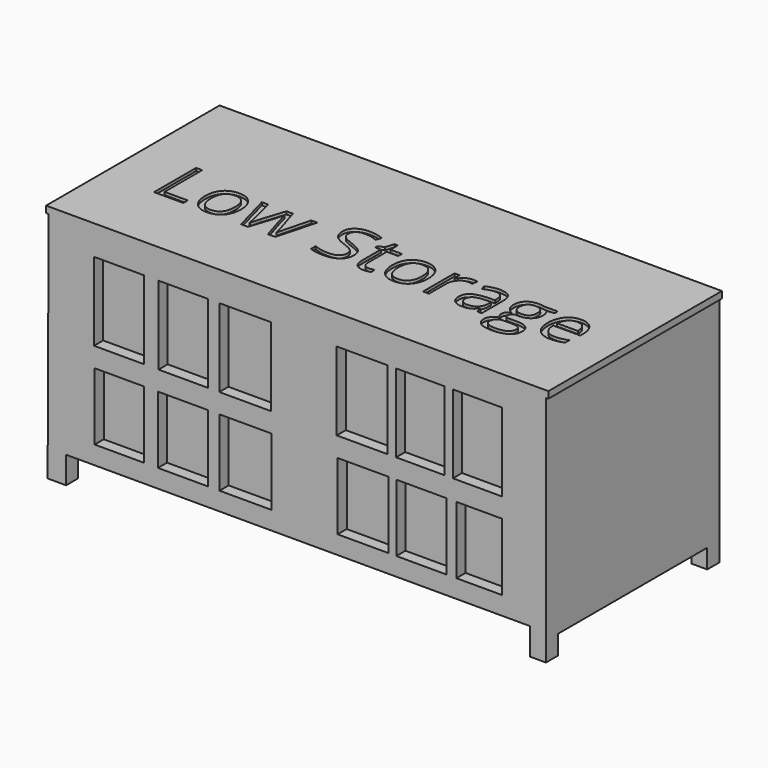
from build123d import *

# Parameters (mm, degrees)
F0_W         = 1117.6
F0_H         = 482.6
F1_DEPTH     = 533.4
F2_W         = 1032.1243926883
F2_H         = 59.8569884896
F3_DEPTH     = 482.601
F4_W         = 415.7167449594
F4_H         = 42.7146777511
F5_DEPTH     = 1117.601
F6_W         = 111.7840632796
F6_H         = 174.2089092731
F6_W_2       = 110.3323251009
F6_W_3       = 114.6875321865
F6_W_4       = 108.8805794716
F6_W_5       = 107.4288487434
F6_W_6       = 113.2358312607
F6_H_2       = 149.5293006301
F6_W_7       = 111.784055829
F6_W_8       = 116.139292717
F6_W_9       = 101.6219258308
F6_W_10      = 111.7841005325
F6_W_11      = 113.235771656
F7_DEPTH     = 25.4
F8_TEXT_SIZE = 163.7518405914
F9_DEPTH     = 6.35
F10_W        = 5.4096342087
F10_H        = 518.5263156891
F11_DEPTH    = 482.6010001


# Not quite as in the source:
# - a length typed as a fraction of an inch, garbled in the dataset ("3 / 203.2 mm" for 3/8 in), is restored
# - Text() gives the source's letters only with a copy of the font that has no kerning and outlines rounded to 1/6400 em; it was checked with that copy


with BuildPart() as f1:
    # F0 (on Top) → F1 (new body)
    with BuildSketch(Plane.XY):
        with Locations((558.8, 241.3)):
            Rectangle(F0_W, F0_H)
    extrude(amount=F1_DEPTH)

    # F2 (on face) → F3 (cut, through all)
    with BuildSketch(Plane.XZ):
        with Locations((560.7183612883, 29.9284942448)):
            Rectangle(F2_W, F2_H)
    extrude(amount=-F3_DEPTH, mode=Mode.SUBTRACT)

    # F4 (on face) → F5 (cut, through all)
    with BuildSketch(Plane.YZ.offset(1117.6)):
        with Locations((240.7026998699, 21.3573388755)):
            Rectangle(F4_W, F4_H)
    extrude(amount=-F5_DEPTH, mode=Mode.SUBTRACT)

    # F6 (on face) → F7 (cut)
    with BuildSketch(Plane.XZ):
        with Locations((162.4746061862, 380.6616812944)):
            Rectangle(F6_W, F6_H)
        with Locations((305.4711148143, 380.6616812944)):
            Rectangle(F6_W_2, F6_H)
        with Locations((442.6606446505, 380.6616812944)):
            Rectangle(F6_W_3, F6_H)
        with Locations((959.4804644585, 380.6616812944)):
            Rectangle(F6_W_4, F6_H)
        with Locations((832.4531316757, 380.6616812944)):
            Rectangle(F6_W_5, F6_H)
        with Locations((703.2481729984, 380.6616812944)):
            Rectangle(F6_W_6, F6_H)
        with Locations((163.2005050778, 175.2402968705)):
            Rectangle(F6_W_2, F6_H_2)
        with Locations((304.7452494502, 175.2402968705)):
            Rectangle(F6_W_7, F6_H_2)
        with Locations((443.9914307247, 175.2402968705)):
            Rectangle(F6_W_8, F6_H_2)
        with Locations((963.7147268901, 175.2402968705)):
            Rectangle(F6_W_9, F6_H_2)
        with Locations((835.2356335769, 175.2402968705)):
            Rectangle(F6_W_10, F6_H_2)
        with Locations((705.3048095355, 175.2402968705)):
            Rectangle(F6_W_11, F6_H_2)
    extrude(amount=-F7_DEPTH, mode=Mode.SUBTRACT)

    # F8 (on face) → F9 (cut)
    with BuildSketch(Plane.XY.offset(533.4)):
        with Locations((98.7801775336, 156.6599458456)):
            Text('Low Storage', F8_TEXT_SIZE, font='Open Sans', text_align=(TextAlign.LEFT, TextAlign.BOTTOM))
    extrude(amount=-F9_DEPTH, mode=Mode.SUBTRACT)

    # F10 (on face) → F11 (cut, through all)
    with BuildSketch(Plane.XZ):
        with Locations((1114.8951828957, 259.2631578445)):
            Rectangle(F10_W, F10_H)
        Polygon((5.6633031927, 518.5263156891), (0, 518.5263156891), (0, 0), (3.4342673607, 0), align=None)
    extrude(amount=-F11_DEPTH, mode=Mode.SUBTRACT)


solid = f1.part
